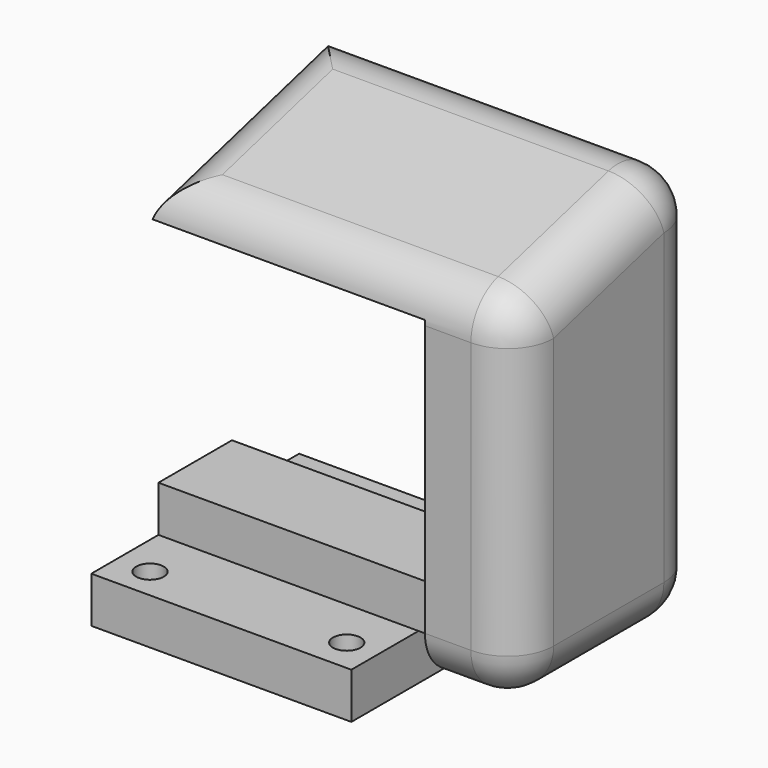
from build123d import *

# Parameters (mm, degrees)
F0_W          = 28.3
F0_H          = 28.2685337434
F0_R          = 1.5
F1_DEPTH      = 5
F2_W          = 45
F2_H          = 10
F3_DEPTH      = 5
F4_W          = 10
F4_H          = 25
F5_DEPTH      = 35
F7_DEPTH      = 30
F7_DEPTH_BACK = 10
F8_T1_DEPTH   = 51.2903171605
F8_T3_DEPTH   = 50.8819045103
F8_T5_DEPTH   = 44.5915873497
F8_T7_DEPTH   = 15.5291427062
F8_T9_DEPTH   = 33.4838731358
F8_T11_DEPTH  = 29.4646352493
F8_T13_DEPTH  = 15
F8_T15_DEPTH  = 17.5
F8_T20_DEPTH  = 5
F8_T26_DEPTH  = 5
F8_S31_W      = 5
F8_S31_H      = 5
F8_T32_DEPTH  = 5
F8_S37_W      = 5
F8_S37_H      = 5
F8_T38_DEPTH  = 5


# Not quite as in the source:
# - a fillet or chamfer that OpenCascade refuses, or shapes differently, is made with other operations: its cross-section is extruded or revolved along the edge and cut away or added


with BuildPart() as f1:
    # F0 (on Top) → F1 (new body)
    with BuildSketch(Plane.XY):
        Rectangle(F0_W, F0_H)
        with Locations((-10.4845586502, -10.7272564019)):
            Circle(F0_R, mode=Mode.SUBTRACT)
        with Locations((10.7272564019, -10.4845586502)):
            Circle(F0_R, mode=Mode.SUBTRACT)
        with Locations((-10.7272564019, 10.4845586502)):
            Circle(F0_R, mode=Mode.SUBTRACT)
        with Locations((10.4845586502, 10.7272564019)):
            Circle(F0_R, mode=Mode.SUBTRACT)
    extrude(amount=F1_DEPTH)

    # F2 (on face) → F3 (join)
    with BuildSketch(Plane.XY.offset(5)):
        with Locations((8.35, 0)):
            Rectangle(F2_W, F2_H)
    extrude(amount=F3_DEPTH)

    # F4 (on face) → F5 (join)
    with BuildSketch(Plane(origin=(0, 0, 5), x_dir=(1, 0, 0), z_dir=(0, 0, -1))):
        with Locations((25.85, 0)):
            Rectangle(F4_W, F4_H)
    extrude(amount=-F5_DEPTH)

    # F6 (on face) → F7 (join, two sides)
    with BuildSketch(Plane(origin=(20.85, 0, 0), x_dir=(0, -1, 0), z_dir=(-1, 0, 0))) as f7_sk:
        Polygon((-12.5, 50), (-12.5, 40), (12.5, 40), (12.5, 43.3012701892), align=None)
    extrude(amount=F7_DEPTH)
    extrude(f7_sk.sketch, amount=-F7_DEPTH_BACK)

    # F8: fillet of radius 5 on 9 edges, made by hand

    # F8_s2 → F8_t1 (cut)
    with BuildSketch(Plane.YZ.offset(-25.4403171605)):
        with BuildLine():
            ThreePointArc((6.2059047745, 48.3135022672), (10.543807145, 47.4506398373), (12.5, 43.4838731358))
            Line((12.5, 43.4838731358), (12.5, 50))
            Line((12.5, 50), (6.2059047745, 48.3135022672))
        make_face()
    extrude(amount=F8_T1_DEPTH, mode=Mode.SUBTRACT)

    # F8_s4 → F8_t3 (cut)
    with BuildSketch(Plane(origin=(0, -12.911414055, -3.4596029692), x_dir=(1, 0, 0), z_dir=(0, 0.9659258263, 0.2588190451))):
        with BuildLine():
            ThreePointArc((-9.15, -40.0610532507), (-7.6855339059, -43.5965871566), (-4.15, -45.0610532507))
            Line((-4.15, -45.0610532507), (-9.15, -45.0610532507))
            Line((-9.15, -45.0610532507), (-9.15, -40.0610532507))
        make_face()
    extrude(amount=F8_T3_DEPTH, mode=Mode.SUBTRACT)

    # F8_s6 → F8_t5 (cut)
    with BuildSketch(Plane.YZ.offset(-18.7415873497)):
        with BuildLine():
            ThreePointArc((-12.5, 39.4646352493), (-11.4667667015, 42.5084423944), (-8.7940952255, 44.2942643808))
            Line((-8.7940952255, 44.2942643808), (-12.5, 43.3012701892))
            Line((-12.5, 43.3012701892), (-12.5, 39.4646352493))
        make_face()
    extrude(amount=F8_T5_DEPTH, mode=Mode.SUBTRACT)

    # F8_s8 → F8_t7 (cut)
    with BuildSketch(Plane(origin=(0, 2.8685635481, 0.7686292862), x_dir=(1, 0, 0), z_dir=(0, 0.9659258263, 0.2588190451))):
        with BuildLine():
            ThreePointArc((25.85, -45.0610532507), (29.3855339059, -43.5965871566), (30.85, -40.0610532507))
            Line((30.85, -40.0610532507), (30.85, -45.0610532507))
            Line((30.85, -45.0610532507), (25.85, -45.0610532507))
        make_face()
    extrude(amount=F8_T7_DEPTH, mode=Mode.SUBTRACT)

    # F8_s10 → F8_t9 (cut)
    with BuildSketch(Plane.XY.offset(10)):
        with BuildLine():
            ThreePointArc((30.85, 7.5), (29.3855339059, 11.0355339059), (25.85, 12.5))
            Line((25.85, 12.5), (30.85, 12.5))
            Line((30.85, 12.5), (30.85, 7.5))
        make_face()
    extrude(amount=F8_T9_DEPTH, mode=Mode.SUBTRACT)

    # F8_s12 → F8_t11 (cut)
    with BuildSketch(Plane.XY.offset(10)):
        with BuildLine():
            ThreePointArc((25.85, -12.5), (29.3855339059, -11.0355339059), (30.85, -7.5))
            Line((30.85, -7.5), (30.85, -12.5))
            Line((30.85, -12.5), (25.85, -12.5))
        make_face()
    extrude(amount=F8_T11_DEPTH, mode=Mode.SUBTRACT)

    # F8_s14 → F8_t13 (cut)
    with BuildSketch(Plane.XZ.offset(-7.5)):
        with BuildLine():
            ThreePointArc((30.85, 10), (29.3855339059, 6.4644660941), (25.85, 5))
            Line((25.85, 5), (30.85, 5))
            Line((30.85, 5), (30.85, 10))
        make_face()
    extrude(amount=F8_T13_DEPTH, mode=Mode.SUBTRACT)

    # F8_s16 → F8_t15 (cut)
    with BuildSketch(Plane.YZ.offset(8.35)):
        with BuildLine():
            ThreePointArc((12.5, 10), (11.0355339059, 6.4644660941), (7.5, 5))
            Line((7.5, 5), (12.5, 5))
            Line((12.5, 5), (12.5, 10))
        make_face()
        with BuildLine():
            ThreePointArc((-12.5, 10), (-11.0355339059, 6.4644660941), (-7.5, 5))
            Line((-7.5, 5), (-12.5, 5))
            Line((-12.5, 5), (-12.5, 10))
        make_face()
    extrude(amount=F8_T15_DEPTH, mode=Mode.SUBTRACT)


with BuildPart() as f8_tool18:
    # F8_s19 → F8_t20 (new body)
    with BuildSketch(Plane.YZ.offset(25.85)):
        Polygon((7.5, 43.4838731358), (12.5, 43.4838731358), (12.5, 50), (6.2059047745, 48.3135022672), align=None)
    extrude(amount=F8_T20_DEPTH)

    # F8_s21 → F8_t22 (revolve, cut)
    with BuildSketch(Plane(origin=(25.85, 7.5, 43.4838731358), x_dir=(0, -0.608761429, -0.7933533403), z_dir=(0, -0.7933533403, 0.608761429))):
        with BuildLine():
            ThreePointArc((0, -5), (5, 0), (0, 5))
            Line((0, 5), (0, -5))
        make_face()
    revolve(axis=Axis((25.85, 7.5, 43.4838731358), (1, 0, 0)), mode=Mode.SUBTRACT)


with BuildPart() as f1_1:
    add(f1.part)

    # F8_t17: cut F8_tool18
    add(f8_tool18.part, mode=Mode.SUBTRACT)


with BuildPart() as f8_tool24:
    # F8_s25 → F8_t26 (new body)
    with BuildSketch(Plane.YZ.offset(25.85)):
        Polygon((-7.5, 39.4646352493), (-12.5, 39.4646352493), (-12.5, 43.3012701892), (-8.7940952255, 44.2942643808), align=None)
    extrude(amount=F8_T26_DEPTH)

    # F8_s27 → F8_t28 (revolve, cut)
    with BuildSketch(Plane(origin=(25.85, -7.5, 39.4646352493), x_dir=(0, 0.7933533403, -0.608761429), z_dir=(0, -0.608761429, -0.7933533403))):
        with BuildLine():
            ThreePointArc((0, -5), (5, 0), (0, 5))
            Line((0, 5), (0, -5))
        make_face()
    revolve(axis=Axis((25.85, -7.5, 39.4646352493), (1, 0, 0)), mode=Mode.SUBTRACT)


with BuildPart() as f1_2:
    add(f1_1.part)

    # F8_t23: cut F8_tool24
    add(f8_tool24.part, mode=Mode.SUBTRACT)


with BuildPart() as f8_tool30:
    # F8_s31 → F8_t32 (new body)
    with BuildSketch(Plane.XZ.offset(-7.5)):
        with Locations((28.35, 7.5)):
            Rectangle(F8_S31_W, F8_S31_H)
    extrude(amount=-F8_T32_DEPTH)

    # F8_s33 → F8_t34 (revolve, cut)
    with BuildSketch(Plane(origin=(25.85, 7.5, 10), x_dir=(-0.7071067812, 0, 0.7071067812), z_dir=(-0.7071067812, 0, -0.7071067812))):
        with BuildLine():
            ThreePointArc((0, -5), (5, 0), (0, 5))
            Line((0, 5), (0, -5))
        make_face()
    revolve(axis=Axis((25.85, 7.5, 10), (0, 1, 0)), mode=Mode.SUBTRACT)


with BuildPart() as f1_3:
    add(f1_2.part)

    # F8_t29: cut F8_tool30
    add(f8_tool30.part, mode=Mode.SUBTRACT)


with BuildPart() as f8_tool36:
    # F8_s37 → F8_t38 (new body)
    with BuildSketch(Plane.XY.offset(10)):
        with Locations((28.35, -10)):
            Rectangle(F8_S37_W, F8_S37_H)
    extrude(amount=-F8_T38_DEPTH)

    # F8_s39 → F8_t40 (revolve, cut)
    with BuildSketch(Plane(origin=(25.85, -7.5, 10), x_dir=(-0.7071067812, 0.7071067812, 0), z_dir=(-0.7071067812, -0.7071067812, 0))):
        with BuildLine():
            ThreePointArc((0, -5), (5, 0), (0, 5))
            Line((0, 5), (0, -5))
        make_face()
    revolve(axis=Axis((25.85, -7.5, 10), (0, 0, -1)), mode=Mode.SUBTRACT)


with BuildPart() as f1_4:
    add(f1_3.part)

    # F8_t35: cut F8_tool36
    add(f8_tool36.part, mode=Mode.SUBTRACT)


solid = f1_4.part
